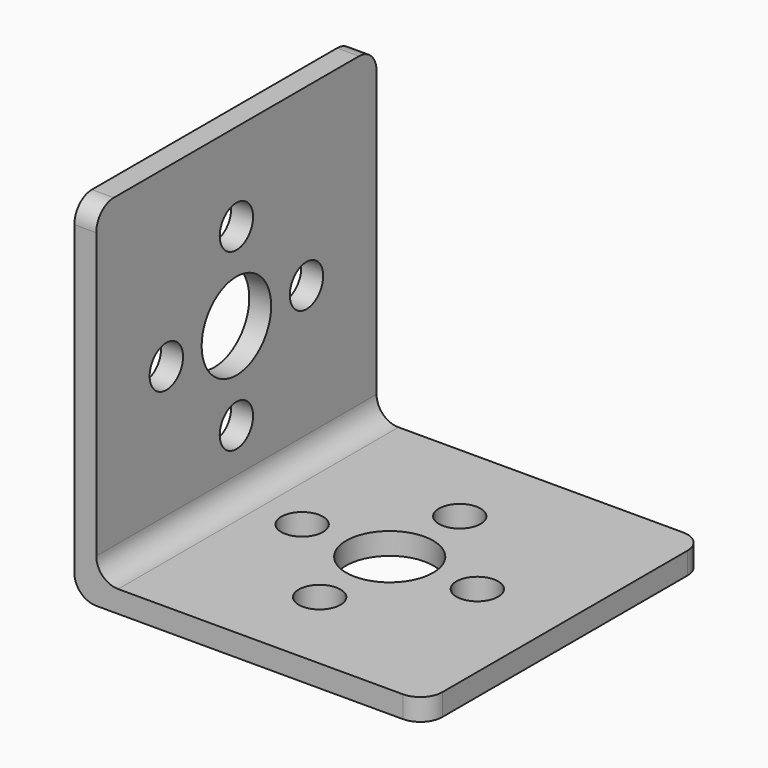
from build123d import *

# Parameters (mm, degrees)
F0_W     = 32
F0_H     = 32
F0_R     = 1.905
F0_R_2   = 3.96875
F1_DEPTH = 2
F2_W     = 2
F2_H     = 32
F3_DEPTH = 30
F4_R     = 3.96875
F4_R_2   = 1.905
F5_DEPTH = 2
F6_R     = 2


# Not quite as in the source:
# - a feature names something its author has since deleted; it is built from what else it names


with BuildPart() as f1:
    # F0 (on Top) → F1 (new body)
    with BuildSketch(Plane.XY):
        with Locations((-16, 16)):
            Rectangle(F0_W, F0_H)
        with Locations((-16, 8)):
            Circle(F0_R, mode=Mode.SUBTRACT)
        with Locations((-24, 16)):
            Circle(F0_R, mode=Mode.SUBTRACT)
        with Locations((-16, 16)):
            Circle(F0_R_2, mode=Mode.SUBTRACT)
        with Locations((-8, 16)):
            Circle(F0_R, mode=Mode.SUBTRACT)
        with Locations((-16, 24)):
            Circle(F0_R, mode=Mode.SUBTRACT)
    extrude(amount=F1_DEPTH)

    # F2 (on face) → F3 (join)
    with BuildSketch(Plane.XY.offset(2)):
        with Locations((-31, 16)):
            Rectangle(F2_W, F2_H)
    extrude(amount=F3_DEPTH)

    # F4 (on face) → F5 (cut, through all)
    with BuildSketch(Plane(origin=(-32, 0, 0), x_dir=(0, -1, 0), z_dir=(-1, 0, 0))):
        with Locations((-16, 16)):
            Circle(F4_R)
        with Locations((-16, 24)):
            Circle(F4_R_2)
        with Locations((-24, 16)):
            Circle(F4_R_2)
        with Locations((-16, 8)):
            Circle(F4_R_2)
        with Locations((-8, 16)):
            Circle(F4_R_2)
    extrude(amount=-F5_DEPTH, mode=Mode.SUBTRACT)

    # F6
    f6_edges = [f1.edges().sort_by_distance(p)[0] for p in [
        (-31, 0, 32),
        (-31, 32, 32),
        (0, 0, 1),
        (0, 32, 1),
        (-30, 16, 2),
        (-32, 16, 0),
    ]]
    fillet(f6_edges, radius=F6_R)


solid = f1.part
